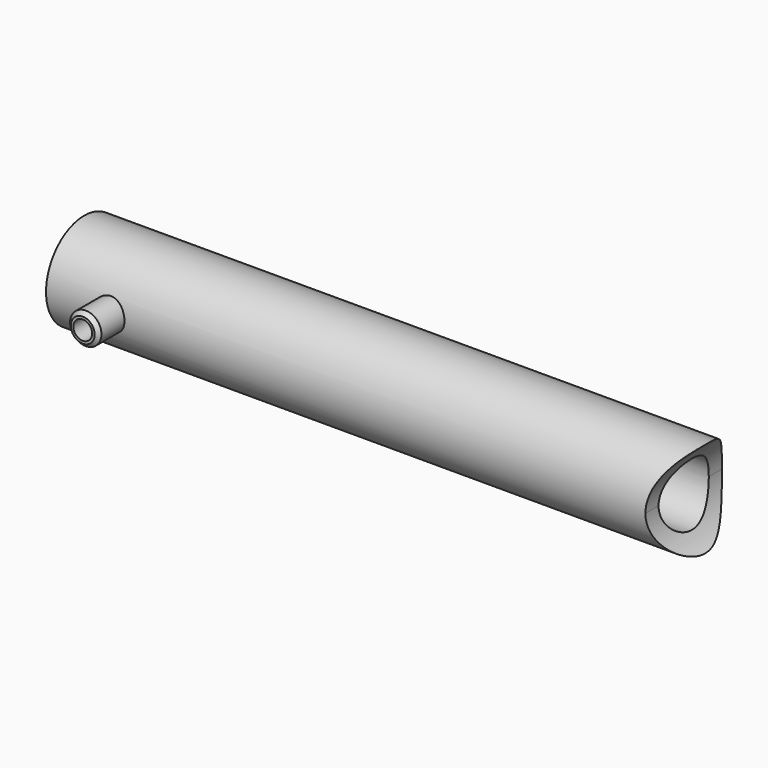
from build123d import *
from build123d import SkipClean  # not in build123d's __all__

# Parameters (mm, degrees)
F0_R      = 12.5
F0_R_2    = 7.5
F1_DEPTH  = 64
F2_R      = 38.1
F2_R_2    = 25
F3_DEPTH  = 100
F4_DEPTH  = 50
F5_SIZE   = 3
F6_R      = 25
F7_DEPTH  = 200
F8_R      = 7.5
F9_DEPTH  = 50
F10_DEPTH = 100
F11_R     = 7.5
F12_DEPTH = 50
F13_DEPTH = 250


with BuildPart() as f1:
    # F0 (on Front) → F1 (new body)
    with BuildSketch(Plane.XZ):
        Circle(F0_R)
        Circle(F0_R_2, mode=Mode.SUBTRACT)
    extrude(amount=F1_DEPTH)

    # F2 (on Right) → F3 (join)
    with BuildSketch(Plane.YZ):
        Circle(F2_R)
        Circle(F2_R_2, mode=Mode.SUBTRACT)
    extrude(amount=F3_DEPTH)

    # F2 (on Right) → F4 (join)
    with BuildSketch(Plane.YZ):
        Circle(F2_R)
        Circle(F2_R_2, mode=Mode.SUBTRACT)
    extrude(amount=-F4_DEPTH)

    # F5
    f5_edges = [f1.edges().sort_by_distance(p)[0] for p in [
        (-12.5, -64, 0),
    ]]
    chamfer(f5_edges, length=F5_SIZE)

    # F6 (on face) → F7 (cut)
    with BuildSketch(Plane(origin=(-50, 0, 0), x_dir=(0, -1, 0), z_dir=(-1, 0, 0))):
        Circle(F6_R)
    extrude(amount=-F7_DEPTH, mode=Mode.SUBTRACT)

    # F8 (on face) → F9 (cut)
    with BuildSketch(Plane.XZ.offset(64)):
        Circle(F8_R)
    extrude(amount=-F9_DEPTH, mode=Mode.SUBTRACT)

    # F10 (add): a face of the model
    f10_faces = [f1.faces().sort_by_distance(p)[0] for p in [
        (100, -37.0223692655, 0),
    ]]
    with SkipClean():  # cleaning this boolean's faces spoils the solid; the shape is the same uncleaned
        extrude(f10_faces, amount=F10_DEPTH)

    # F11 (on face) → F12 (cut)
    with BuildSketch(Plane.XZ.offset(64)):
        Circle(F11_R)
    with SkipClean():  # cleaning this boolean's faces spoils the solid; the shape is the same uncleaned
        extrude(amount=-F12_DEPTH, mode=Mode.SUBTRACT)

    # F13 (add): a face of the model
    f13_faces = [f1.faces().sort_by_distance(p)[0] for p in [
        (200, -37.0223692655, 0),
    ]]
    extrude(f13_faces, amount=F13_DEPTH)

    # F14 (on Top) → F15 (revolve, cut)
    with BuildSketch(Plane.XY):
        Polygon((455.1408666709, 52.4849742776), (427.6145875454, 51.9348941743), (427.6145875454, -50.6588555872), (455.1408666709, -51.4342445287), align=None)
    with SkipClean():  # cleaning this boolean's faces spoils the solid; the shape is the same uncleaned
        revolve(axis=Axis((478.6976158619, 0.4289562068, 0), (0, -1, 0)), mode=Mode.SUBTRACT)


solid = f1.part
